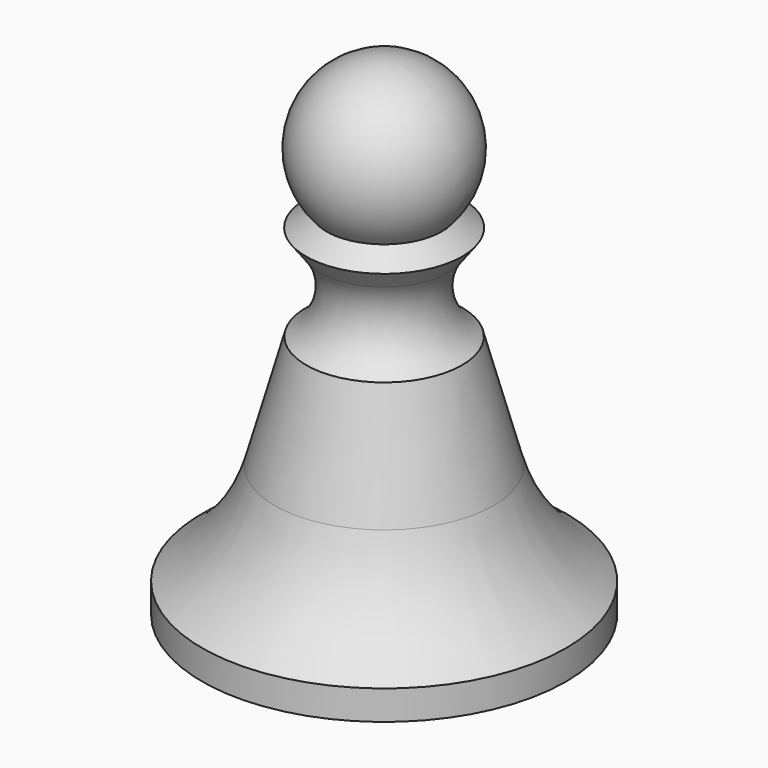
from build123d import *


# Not quite as in the source:
# - a fillet or chamfer that OpenCascade refuses, or shapes differently, is made with other operations: its cross-section is extruded or revolved along the edge and cut away or added


with BuildPart() as f1:
    # F0 (on Front) → F1 (revolve)
    with BuildSketch(Plane.XZ):
        with BuildLine():
            Line((0, 38.5912625485), (0, 0))
            Line((0, 0), (19.7524651885, 0))
            Line((19.7524651885, 0), (19.7524651885, 3.1980082858))
            Line((19.7524651885, 3.1980082858), (14.1919255257, 5.8136251755))
            Line((14.1919255257, 5.8136251755), (8.4569835516, 26.5488596043))
            ThreePointArc((8.4569835516, 26.5488596043), (5.8902046524, 30.3760769017), (6.9375761897, 34.8637220549))
            Line((6.9375761897, 34.8637220549), (8.4767341614, 36.9339473546))
            Line((8.4767341614, 36.9339473546), (6.2475829585, 38.5912625485))
            ThreePointArc((6.2475829585, 38.5912625485), (7.9366897799, 47.9479775999), (0, 53.183448328))
            Line((0, 53.183448328), (0, 38.5912625485))
        make_face()
    revolve(axis=Axis((0, 0, 19.2956312742), (0, 0, 1)))

    # F2: fillet of radius 19.7282149364 on 1 edges, made by hand

    # F2_s1 → F2_t2 (revolve)
    with BuildSketch(Plane.XZ):
        with BuildLine():
            ThreePointArc((19.7524651885, 3.1980082858), (14.8303095618, 8.0151476836), (11.8639351327, 14.2306984022))
            Line((11.8639351327, 14.2306984022), (11.4836480923, 14.1255187807))
            Line((11.4836480923, 14.1255187807), (13.8116384853, 5.708445554))
            Line((13.8116384853, 5.708445554), (14.0239794459, 5.4565886226))
            ThreePointArc((14.0239794459, 5.4565886226), (16.8042492773, 4.1487801778), (19.5299487493, 2.872174862))
            Line((19.5299487493, 2.872174862), (19.7524651885, 3.1980082858))
        make_face()
    revolve(axis=Axis((0, 0, 5.8136251755), (0, 0, 1)))


solid = f1.part
